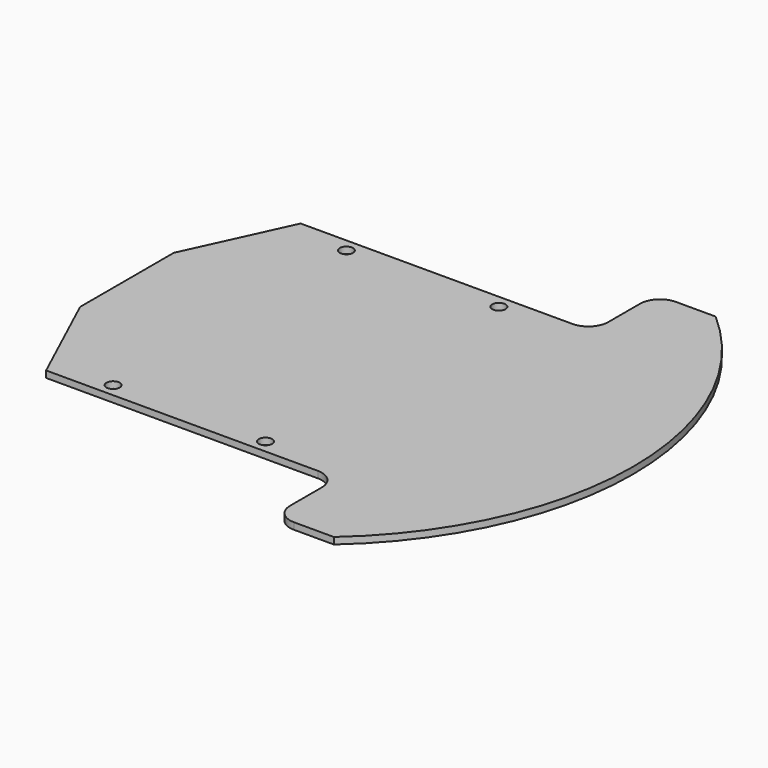
from build123d import *

# Parameters (mm, degrees)
F0_R     = 1
F1_DEPTH = 1
F2_R     = 3


with BuildPart() as f1:
    # F0 (on Top) → F1 (new body)
    with BuildSketch(Plane.XY):
        with BuildLine():
            Line((24, 24), (0, 24))
            Line((0, 24), (-20, 24))
            Line((-20, 24), (-27, 8.8345631957))
            Line((-27, 8.8345631957), (-27, 0))
            Line((-27, 0), (-27, -8.8345631957))
            Line((-27, -8.8345631957), (-20, -24))
            Line((-20, -24), (0, -24))
            Line((0, -24), (24, -24))
            Line((24, -24), (24, -36))
            Line((24, -36), (33, -36))
            ThreePointArc((33, -36), (49.3356561573, 0), (33, 36))
            Line((33, 36), (24, 36))
            Line((24, 36), (24, 24))
        make_face()
        with Locations((-11.5, -22)):
            Circle(F0_R, mode=Mode.SUBTRACT)
        with Locations((11.5, -22)):
            Circle(F0_R, mode=Mode.SUBTRACT)
        with Locations((-11.5, 22)):
            Circle(F0_R, mode=Mode.SUBTRACT)
        with Locations((11.5, 22)):
            Circle(F0_R, mode=Mode.SUBTRACT)
    extrude(amount=F1_DEPTH)

    # F2
    f2_edges = [f1.edges().sort_by_distance(p)[0] for p in [
        (24, -24, 0.5),
        (24, -36, 0.5),
        (24, 24, 0.5),
        (24, 36, 0.5),
    ]]
    fillet(f2_edges, radius=F2_R)


solid = f1.part
